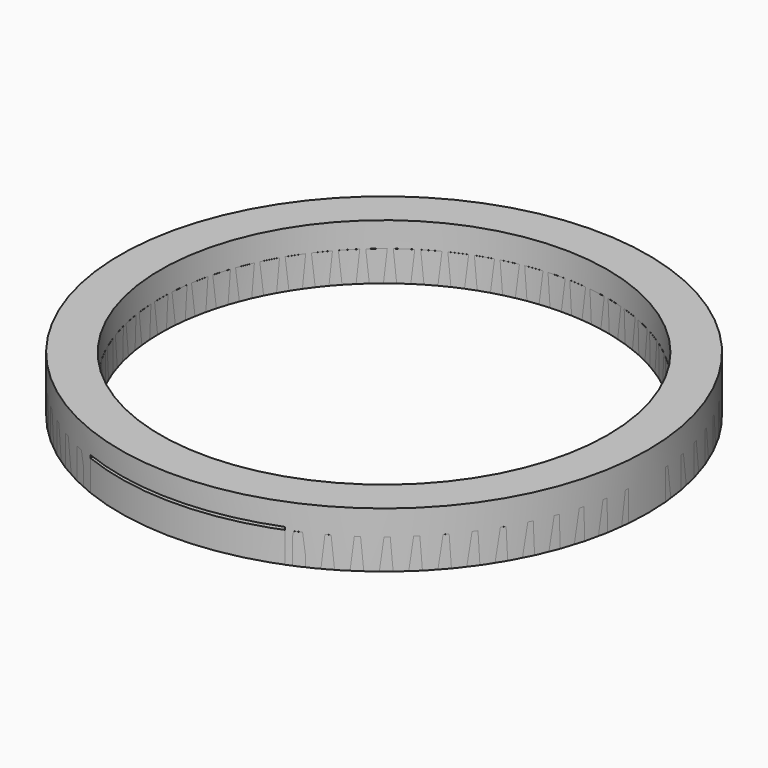
from build123d import *

# Parameters (mm, degrees)
F0_R     = 9.5
F0_R_2   = 8.05
F1_DEPTH = 1.1
F2_DEPTH = 2
F4_DEPTH = 1.2
F5_SCALE = 3


with BuildPart() as f1:
    # F0 (on Top) → F1 (new body)
    with BuildSketch(Plane.XY):
        Circle(F0_R)
        Circle(F0_R_2, mode=Mode.SUBTRACT)
    extrude(amount=F1_DEPTH)


with BuildPart() as f2:
    # F0 (on Top) → F2 (new body)
    with BuildSketch(Plane.XY):
        Circle(F0_R)
        Circle(F0_R_2, mode=Mode.SUBTRACT)
    extrude(amount=F2_DEPTH)

    # F3 (on face) → F4 (cut)
    with BuildSketch(Plane(origin=(0, 0, 0), x_dir=(1, 0, 0), z_dir=(0, 0, -1))):
        with BuildLine():
            ThreePointArc((3.5, 8.8317608663), (0, 9.5), (-3.5, 8.8317608663))
            Line((-3.5, 8.8317608663), (-3.5, 7.249310312))
            ThreePointArc((-3.5, 7.249310312), (0, 8.05), (3.5, 7.249310312))
            Line((3.5, 7.249310312), (3.5, 8.8317608663))
        make_face()
    extrude(amount=-F4_DEPTH, mode=Mode.SUBTRACT)


with BuildPart() as f1_1:
    # F5: moved
    add(f1.part.scale(F5_SCALE))


with BuildPart() as f2_1:
    # F5: moved
    add(f2.part.scale(F5_SCALE))


solid = Compound([f1_1.part, f2_1.part])
